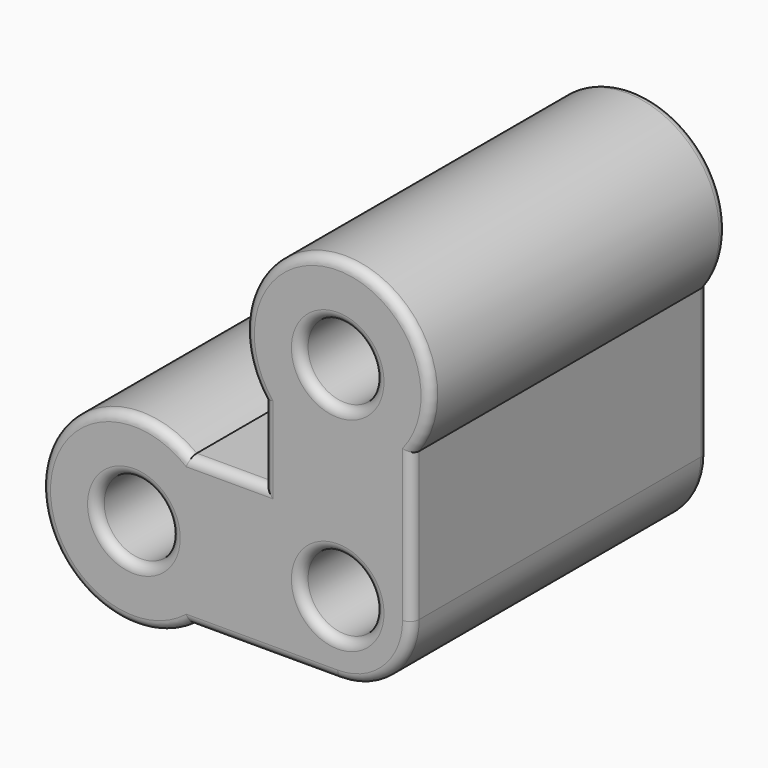
from build123d import *

# Parameters (mm, degrees)
F0_R     = 6.35
F1_DEPTH = 63.5
F2_R     = 1.5875


# Not quite as in the source:
# - a feature names something its author has since deleted; it is built from what else it names


with BuildPart() as f1:
    # F0 (on Front) → F1 (new body)
    with BuildSketch(Plane.XZ):
        with BuildLine():
            Line((-12.7, 12.7), (-25.4, 12.7))
            ThreePointArc((-25.4, 12.7), (-50.8, 0), (-25.4, -12.7))
            Line((-25.4, -12.7), (0, -12.7))
            ThreePointArc((0, -12.7), (8.9802561211, -8.9802561211), (12.7, 0))
            Line((12.7, 0), (12.7, 25.4))
            ThreePointArc((12.7, 25.4), (0, 50.8), (-12.7, 25.4))
            Line((-12.7, 25.4), (-12.7, 12.7))
        make_face()
        with Locations((-34.925, 0)):
            Circle(F0_R, mode=Mode.SUBTRACT)
        Circle(F0_R, mode=Mode.SUBTRACT)
        with Locations((0, 34.925)):
            Circle(F0_R, mode=Mode.SUBTRACT)
    extrude(amount=F1_DEPTH)

    # F2
    f2_edges = [f1.edges().sort_by_distance(p)[0] for p in [
        (-12.7, -63.5, 19.05),
        (-19.05, -63.5, 12.7),
        (-50.8, -63.5, 0),
        (-12.7, -63.5, -12.7),
        (8.980256, -63.5, -8.980256),
        (12.7, -63.5, 12.7),
        (0, -63.5, 50.8),
        (-41.275, -63.5, 0),
        (-6.35, -63.5, 0),
        (-6.35, -63.5, 34.925),
        (-12.7, 0, 19.05),
        (-19.05, 0, 12.7),
        (-50.8, 0, 0),
        (-12.7, 0, -12.7),
        (8.980256, 0, -8.980256),
        (12.7, 0, 12.7),
        (0, 0, 50.8),
        (-41.275, 0, 0),
        (-6.35, 0, 0),
        (-6.35, 0, 34.925),
    ]]
    fillet(f2_edges, radius=F2_R)


solid = f1.part
